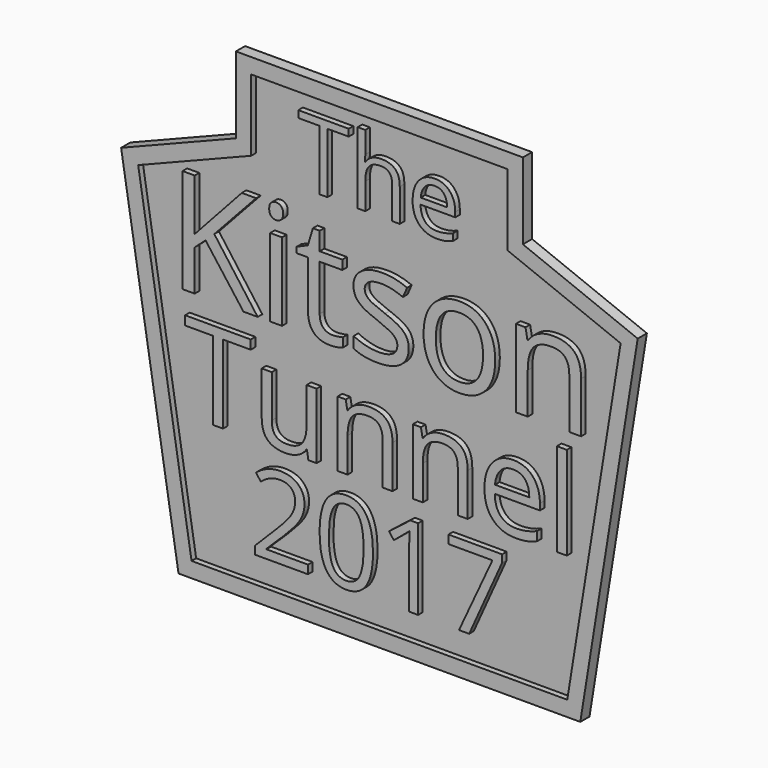
from build123d import *

# Parameters (mm, degrees)
F1_DEPTH       = 3
F2_TEXT_SIZE   = 76.1299148672
F2_TEXT_SIZE_2 = 64.0662086773
F2_TEXT_SIZE_3 = 59.0904727205
F2_TEXT_SIZE_4 = 49.200312831
F3_DEPTH       = 3
F5_DEPTH       = 3


# Not quite as in the source:
# - Text() gives the source's letters only with a copy of the font that has no kerning and outlines rounded to 1/6400 em; it was checked with that copy


with BuildPart() as f1:
    # F0 (on Front) → F1 (new body)
    with BuildSketch(Plane.XZ):
        Polygon((-30, 186.1335635185), (0, 0), (210, 0), (240, 186.1335635185), (180, 210), (180, 250), (105, 250), (30, 250), (30, 210), align=None)
    extrude(amount=F1_DEPTH)

    # F2 (on face) → F3 (join)
    with BuildSketch(Plane.XZ.offset(3)):
        with Locations((-5.3467430102, 131.5261237106)):
            Text('Kitson', F2_TEXT_SIZE, font='Open Sans', text_align=(TextAlign.LEFT, TextAlign.BOTTOM))
        with Locations((2.8944799206, 74.2214541068)):
            Text('Tunnel', F2_TEXT_SIZE_2, font='Open Sans', text_align=(TextAlign.LEFT, TextAlign.BOTTOM))
        with Locations((37.0182577123, 21.6477564586)):
            Text('2017', F2_TEXT_SIZE_3, font='Open Sans', text_align=(TextAlign.LEFT, TextAlign.BOTTOM))
        with Locations((62.1803527393, 198.4492974553)):
            Text('The', F2_TEXT_SIZE_4, font='Open Sans', text_align=(TextAlign.LEFT, TextAlign.BOTTOM))
    extrude(amount=F3_DEPTH)

    # F4 (on face) → F5 (join)
    with BuildSketch(Plane.XZ.offset(3)):
        Polygon((180, 250), (30, 250), (30, 210), (-30, 186.1335635185), (0, 0), (210, 0), (240, 186.1335635185), (180, 210), align=None)
        Polygon((38, 204.5725258614), (38, 242), (172, 242), (172, 204.5725258614), (231.0809101248, 181.0716793821), (203.18615389, 8), (6.81384611, 8), (-21.0809101248, 181.0716793821), align=None, mode=Mode.SUBTRACT)
    extrude(amount=F5_DEPTH)


solid = f1.part
